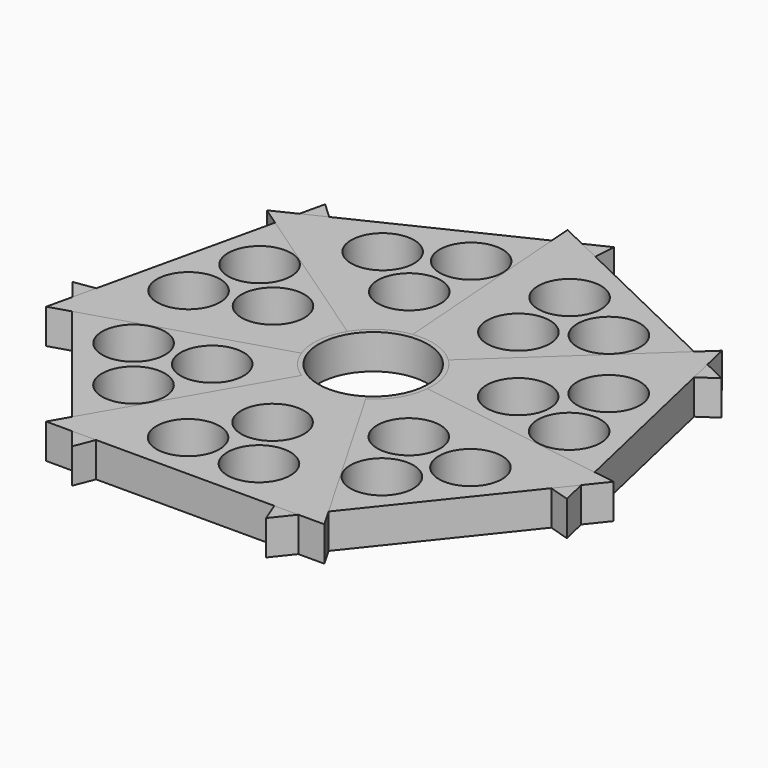
from build123d import *

# Parameters (mm, degrees)
F0_R     = 12.5
F1_DEPTH = 7
F3_DEPTH = 7
F4_SIZE2 = 1
F4_SIZE  = 0.5773502692
F5_SIZE2 = 1
F5_SIZE  = 0.5773502692
F7_D     = 12.7
F8_COUNT = 7
F10_D    = 22
F10_2_D  = 22
F10_3_D  = 22
F10_4_D  = 22
F10_5_D  = 22
F10_6_D  = 22
F10_7_D  = 22


# Not quite as in the source:
# - a feature names something its author has since deleted; it is built from what else it names


with BuildPart() as f1:
    # F0 (on Top) → F1 (new body)
    with BuildSketch(Plane.XY):
        Circle(F0_R)
    extrude(amount=F1_DEPTH)

    # F2 (on Top) + F0 (on Top) → F3 (join)
    with BuildSketch(Plane.XY):
        Polygon((-28.0327634543, -47.4243392048), (28.0828249826, -47.4243392048), (0.0250307641, 1.1731859299), align=None)
    with BuildSketch(Plane.XY):
        Circle(F0_R)
    extrude(amount=F3_DEPTH)

    # F4
    f4_edges = [f1.edges().sort_by_distance(p)[0] for p in [
        (-0.021701, 12.499981, 7),
    ]]
    f4_side = f1.faces().sort_by_distance((0.018297, -23.813654, 7))[0]
    chamfer(f4_edges, length=F4_SIZE, length2=F4_SIZE2, reference=f4_side)

    # F5
    f5_edges = [f1.edges().sort_by_distance(p)[0] for p in [
        (-0.021701, 12.499981, 0),
    ]]
    f5_side = f1.faces().sort_by_distance((0.018297, -23.813654, 0))[0]
    chamfer(f5_edges, length=F5_SIZE, length2=F5_SIZE2, reference=f5_side)

    # F7 (through all)
    with Locations(Plane(origin=(0, 0, 0), x_dir=(1, 0, 0), z_dir=(0, 0, -1))):
        with Locations((0, 25.3569102192), (7.1490397082, 37.7394102192), (-7.1490397082, 37.7394102192)):
            Hole(F7_D / 2)


with BuildPart() as f8_1:
    # F8: instance of F1
    add(f1.part.rotate(Axis((0, 0, 0), (0, 0, -1)), 1 * 360 / F8_COUNT))

    # F10#2 (through all)
    with Locations(Plane(origin=(0, 0, 0), x_dir=(1, 0, 0), z_dir=(0, 0, -1))):
        with Locations((0, 0)):
            Hole(F10_2_D / 2)


with BuildPart() as f8_2:
    # F8: instance of F1
    add(f1.part.rotate(Axis((0, 0, 0), (0, 0, -1)), 2 * 360 / F8_COUNT))

    # F10#3 (through all)
    with Locations(Plane(origin=(0, 0, 0), x_dir=(1, 0, 0), z_dir=(0, 0, -1))):
        with Locations((0, 0)):
            Hole(F10_3_D / 2)


with BuildPart() as f8_3:
    # F8: instance of F1
    add(f1.part.rotate(Axis((0, 0, 0), (0, 0, -1)), 3 * 360 / F8_COUNT))

    # F10#4 (through all)
    with Locations(Plane(origin=(0, 0, 0), x_dir=(1, 0, 0), z_dir=(0, 0, -1))):
        with Locations((0, 0)):
            Hole(F10_4_D / 2)


with BuildPart() as f8_4:
    # F8: instance of F1
    add(f1.part.rotate(Axis((0, 0, 0), (0, 0, -1)), 4 * 360 / F8_COUNT))

    # F10#5 (through all)
    with Locations(Plane(origin=(0, 0, 0), x_dir=(1, 0, 0), z_dir=(0, 0, -1))):
        with Locations((0, 0)):
            Hole(F10_5_D / 2)


with BuildPart() as f8_5:
    # F8: instance of F1
    add(f1.part.rotate(Axis((0, 0, 0), (0, 0, -1)), 5 * 360 / F8_COUNT))

    # F10#6 (through all)
    with Locations(Plane(origin=(0, 0, 0), x_dir=(1, 0, 0), z_dir=(0, 0, -1))):
        with Locations((0, 0)):
            Hole(F10_6_D / 2)


with BuildPart() as f8_6:
    # F8: instance of F1
    add(f1.part.rotate(Axis((0, 0, 0), (0, 0, -1)), 6 * 360 / F8_COUNT))

    # F10#7 (through all)
    with Locations(Plane(origin=(0, 0, 0), x_dir=(1, 0, 0), z_dir=(0, 0, -1))):
        with Locations((0, 0)):
            Hole(F10_7_D / 2)


with BuildPart() as f1_1:
    add(f1.part)

    # F10 (through all)
    with Locations(Plane(origin=(0, 0, 0), x_dir=(1, 0, 0), z_dir=(0, 0, -1))):
        with Locations((0, 0)):
            Hole(F10_D / 2)


solid = Compound([f8_1.part, f8_2.part, f8_3.part, f8_4.part, f8_5.part, f8_6.part, f1_1.part])
